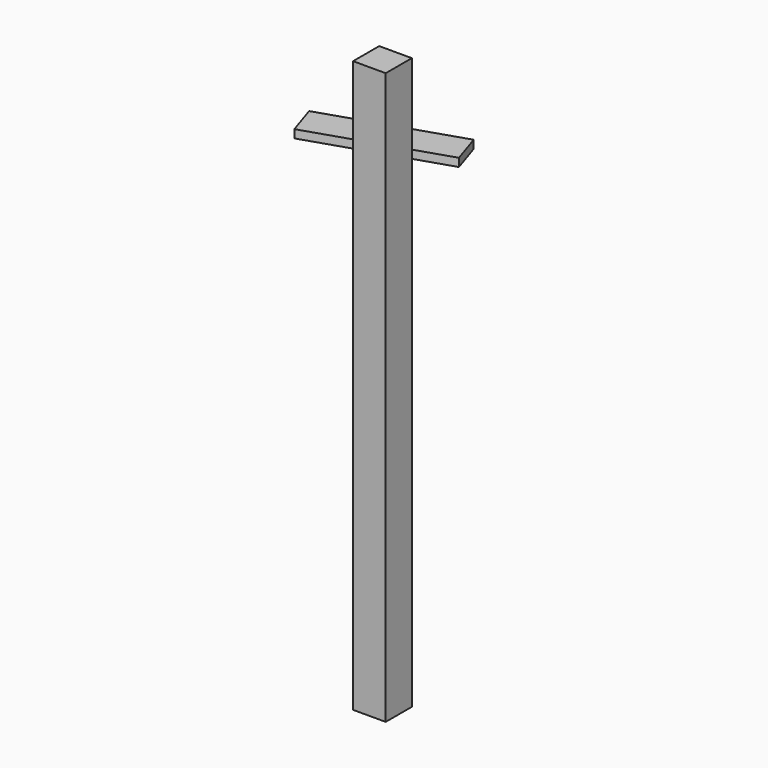
from build123d import *

# Parameters (mm, degrees)
F0_W      = 200
F0_H      = 200
F1_DEPTH  = 3000
F3_DEPTH  = 50
F4_DEPTH  = 500
F5_W      = 90
F5_H      = 108.5
F5_R      = 6
F6_DEPTH  = 2.5
F7_W      = 90
F7_H      = 2.5
F8_DEPTH  = 96
F9_R      = 6
F10_DEPTH = 25
F11_R     = 10
F12_DEPTH = 3
F14_DEPTH = 5
F15_R     = 10
F16_DEPTH = 3
F18_DEPTH = 5
F20_DEPTH = 5
F22_DEPTH = 5


with BuildPart() as f1:
    # F0 (on Top) → F1 (new body)
    with BuildSketch(Plane.XY):
        Rectangle(F0_W, F0_H)
    extrude(amount=F1_DEPTH)

    # F4 (add): a face of the model
    f4_faces = [f1.faces().sort_by_distance(p)[0] for p in [
        (0, 0, 3000),
    ]]
    extrude(f4_faces, amount=F4_DEPTH)


with BuildPart() as f3:
    # F2 (on face) → F3 (new body)
    with BuildSketch(Plane.XY.offset(3000)):
        Polygon((-541.1982426134, 114.3653346673), (-479.3948437385, -75.8459685917), (-100, 47.4268887881), (-100, 100), (61.803398875, 100), (321.2412034368, 184.2964526496), (259.4378045618, 374.5077559086), align=None)
    extrude(amount=-F3_DEPTH)


with BuildPart() as f6:
    # F5 (on face) → F6 (new body)
    with BuildSketch(Plane(origin=(0, 100, 0), x_dir=(-1, 0, 0), z_dir=(0, 1, 0))):
        with Locations((40, 3053.461101532)):
            Rectangle(F5_W, F5_H)
        with Locations((10, 3024.211101532)):
            Circle(F5_R, mode=Mode.SUBTRACT)
        with Locations((70, 3024.211101532)):
            Circle(F5_R, mode=Mode.SUBTRACT)
        with Locations((40, 3092.711101532)):
            Circle(F5_R, mode=Mode.SUBTRACT)
    extrude(amount=F6_DEPTH)

    # F7 (on face) → F8 (join)
    with BuildSketch(Plane(origin=(0, 102.5, 0), x_dir=(-1, 0, 0), z_dir=(0, 1, 0))):
        with Locations((40, 3001.461101532)):
            Rectangle(F7_W, F7_H)
    extrude(amount=F8_DEPTH)

    # F9 (on face) → F10 (cut)
    with BuildSketch(Plane.XY.offset(3002.711101532)):
        with Locations((-70, 130.4318457842)):
            Circle(F9_R)
        with Locations((-10, 130.4318457842)):
            Circle(F9_R)
        with Locations((-40, 178.5)):
            Circle(F9_R)
    extrude(amount=-F10_DEPTH, mode=Mode.SUBTRACT)


with BuildPart() as f12:
    # F11 (on face) → F12 (new body)
    with BuildSketch(Plane(origin=(0, 102.5, 0), x_dir=(-1, 0, 0), z_dir=(0, 1, 0))):
        with Locations((10, 3024.211101532)):
            Circle(F11_R)
    extrude(amount=F12_DEPTH)


with BuildPart() as f12b:
    # F11 (on face) → F12, piece 2 (new body)
    with BuildSketch(Plane(origin=(0, 102.5, 0), x_dir=(-1, 0, 0), z_dir=(0, 1, 0))):
        with Locations((70, 3024.211101532)):
            Circle(F11_R)
    extrude(amount=F12_DEPTH)


with BuildPart() as f14:
    # F13 (on face) → F14 (new body)
    with BuildSketch(Plane(origin=(0, 105.5, 0), x_dir=(-1, 0, 0), z_dir=(0, 1, 0))):
        Polygon((18.831995198, 3026.9183499794), (12.0714516691, 3033.2134579633), (3.2394564712, 3030.5062095158), (1.168004802, 3021.5038530845), (7.9285483309, 3015.2087451007), (16.7605435288, 3017.9159935482), align=None)
    extrude(amount=F14_DEPTH)


with BuildPart() as f16:
    # F15 (on face) → F16 (new body)
    with BuildSketch(Plane.XY.offset(3002.711101532)):
        with Locations((-10, 130.4318457842)):
            Circle(F15_R)
    extrude(amount=F16_DEPTH)


with BuildPart() as f16b:
    # F15 (on face) → F16, piece 2 (new body)
    with BuildSketch(Plane.XY.offset(3002.711101532)):
        with Locations((-70, 130.4318457842)):
            Circle(F15_R)
    extrude(amount=F16_DEPTH)


with BuildPart() as f18:
    # F17 (on face) → F18 (new body)
    with BuildSketch(Plane.XY.offset(3005.711101532)):
        Polygon((-69.8552391039, 139.6683157601), (-77.9266371924, 135.1754473857), (-78.0713980885, 125.9389774097), (-70.1447608961, 121.1953758083), (-62.0733628076, 125.6882441827), (-61.9286019115, 134.9247141586), align=None)
    extrude(amount=F18_DEPTH)


with BuildPart() as f20:
    # F19 (on face) → F20 (new body)
    with BuildSketch(Plane.XY.offset(3005.711101532)):
        Polygon((-13.5356847146, 138.9660280492), (-19.1586609993, 131.6369441341), (-15.6229762847, 123.1027618691), (-6.4643152854, 121.8976635192), (-0.8413390007, 129.2267474343), (-4.3770237153, 137.7609296993), align=None)
    extrude(amount=F20_DEPTH)


with BuildPart() as f22:
    # F21 (on face) → F22 (new body)
    with BuildSketch(Plane(origin=(0, 105.5, 0), x_dir=(-1, 0, 0), z_dir=(0, 1, 0))):
        Polygon((64.716681768, 3031.7886922964), (60.7959547825, 3023.424409109), (66.0792730145, 3015.8468183446), (75.283318232, 3016.6335107676), (79.2040452175, 3024.9977939549), (73.9207269855, 3032.5753847194), align=None)
    extrude(amount=F22_DEPTH)


solid = Compound([f1.part, f3.part, f6.part, f12.part, f12b.part, f14.part, f16.part, f16b.part, f18.part, f20.part, f22.part])
